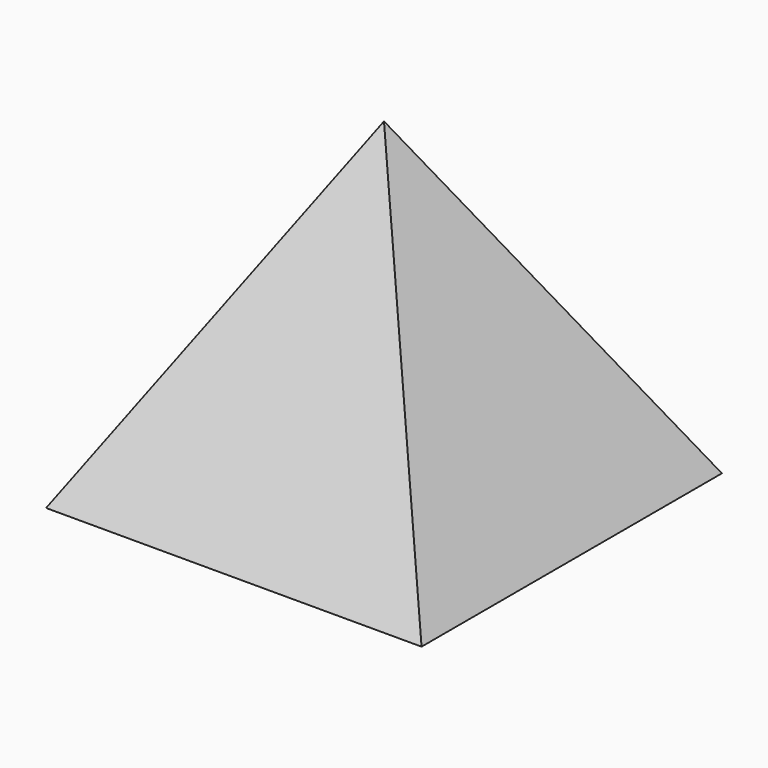
from build123d import *

# Parameters (mm, degrees)
F0_W     = 25.4
F0_H     = 25.4
F1_DEPTH = 37.592
F1_TAPER = 30


with BuildPart() as f1:
    # F0 (on Top) → F1 (new body)
    with BuildSketch(Plane.XY):
        with Locations((-18.514321, 52.058566)):
            Rectangle(F0_W, F0_H)
    extrude(amount=F1_DEPTH, taper=F1_TAPER)


solid = f1.part
